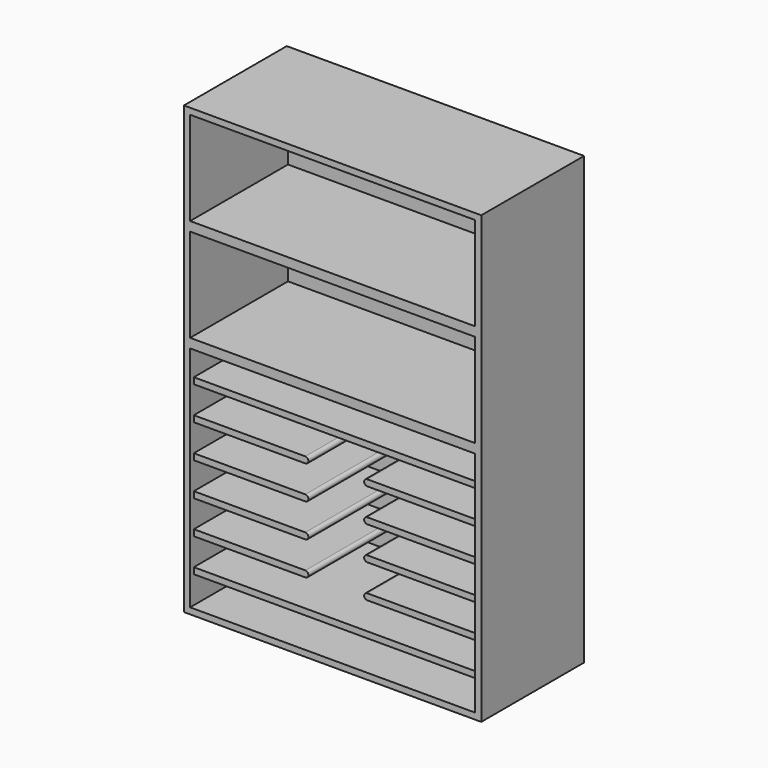
from build123d import *

# Parameters (mm, degrees)
F0_W     = 609.6
F0_H     = 914.4
F1_DEPTH = 263.525
F2_T     = -12.7
F3_W     = 584.2
F3_H     = 19.05
F4_DEPTH = 250.825
F6_DEPTH = 241.3
F7_DEPTH = 241.3


# Not quite as in the source:
# - a feature names something its author has since deleted; it is built from what else it names


with BuildPart() as f1:
    # F0 (on Front) → F1 (new body)
    with BuildSketch(Plane.XZ):
        Rectangle(F0_W, F0_H)
    extrude(amount=F1_DEPTH)

    # F2
    f2_openings = [f1.faces().sort_by_distance(p)[0] for p in [
        (0, -263.525, 0),
    ]]
    offset(amount=F2_T, openings=f2_openings)

    # F3 (on face) → F4 (join)
    with BuildSketch(Plane.XZ.offset(12.7)):
        with Locations((0, 32.385)):
            Rectangle(F3_W, F3_H)
        with Locations((0, 243.205)):
            Rectangle(F3_W, F3_H)
    extrude(amount=F4_DEPTH)

    # F5 (on face) → F6 (join)
    with BuildSketch(Plane.XZ.offset(12.7)):
        Polygon((-63.5, -33.02), (-292.1, -33.02), (-292.1, -45.72), (-63.5, -45.72), (63.5, -45.72), (292.1, -45.72), (292.1, -33.02), (63.5, -33.02), align=None)
    extrude(amount=F6_DEPTH)

    # F5 (on face) → F7 (join)
    with BuildSketch(Plane.XZ.offset(12.7)):
        with BuildLine():
            Line((292.1, -182.88), (292.1, -170.18))
            Line((292.1, -170.18), (63.5, -170.18))
            ThreePointArc((63.5, -170.18), (57.15, -176.53), (63.5, -182.88))
            Line((63.5, -182.88), (292.1, -182.88))
        make_face()
        with BuildLine():
            Line((292.1, -114.3), (292.1, -101.6))
            Line((292.1, -101.6), (63.5, -101.6))
            ThreePointArc((63.5, -101.6), (57.15, -107.95), (63.5, -114.3))
            Line((63.5, -114.3), (292.1, -114.3))
        make_face()
        Polygon((-63.5, -33.02), (-292.1, -33.02), (-292.1, -45.72), (-63.5, -45.72), (63.5, -45.72), (292.1, -45.72), (292.1, -33.02), (63.5, -33.02), align=None)
        with BuildLine():
            Line((-63.5, -170.18), (-292.1, -170.18))
            Line((-292.1, -170.18), (-292.1, -182.88))
            Line((-292.1, -182.88), (-63.5, -182.88))
            ThreePointArc((-63.5, -182.88), (-57.15, -176.53), (-63.5, -170.18))
        make_face()
        with BuildLine():
            Line((-63.5, -101.6), (-292.1, -101.6))
            Line((-292.1, -101.6), (-292.1, -114.3))
            Line((-292.1, -114.3), (-63.5, -114.3))
            ThreePointArc((-63.5, -114.3), (-57.15, -107.95), (-63.5, -101.6))
        make_face()
        with BuildLine():
            Line((-63.5, -238.76), (-292.1, -238.76))
            Line((-292.1, -238.76), (-292.1, -251.46))
            Line((-292.1, -251.46), (-63.5, -251.46))
            ThreePointArc((-63.5, -251.46), (-57.15, -245.11), (-63.5, -238.76))
        make_face()
        with BuildLine():
            Line((292.1, -251.46), (292.1, -238.76))
            Line((292.1, -238.76), (63.5, -238.76))
            ThreePointArc((63.5, -238.76), (57.15, -245.11), (63.5, -251.46))
            Line((63.5, -251.46), (292.1, -251.46))
        make_face()
        with BuildLine():
            Line((292.1, -320.04), (292.1, -307.34))
            Line((292.1, -307.34), (63.5, -307.34))
            ThreePointArc((63.5, -307.34), (57.15, -313.69), (63.5, -320.04))
            Line((63.5, -320.04), (292.1, -320.04))
        make_face()
        with BuildLine():
            Line((-63.5, -307.34), (-292.1, -307.34))
            Line((-292.1, -307.34), (-292.1, -320.04))
            Line((-292.1, -320.04), (-63.5, -320.04))
            ThreePointArc((-63.5, -320.04), (-57.15, -313.69), (-63.5, -307.34))
        make_face()
        Polygon((-63.5, -375.92), (-292.1, -375.92), (-292.1, -388.62), (-63.5, -388.62), (63.5, -388.62), (292.1, -388.62), (292.1, -375.92), (63.5, -375.92), align=None)
    extrude(amount=F7_DEPTH)


solid = f1.part
